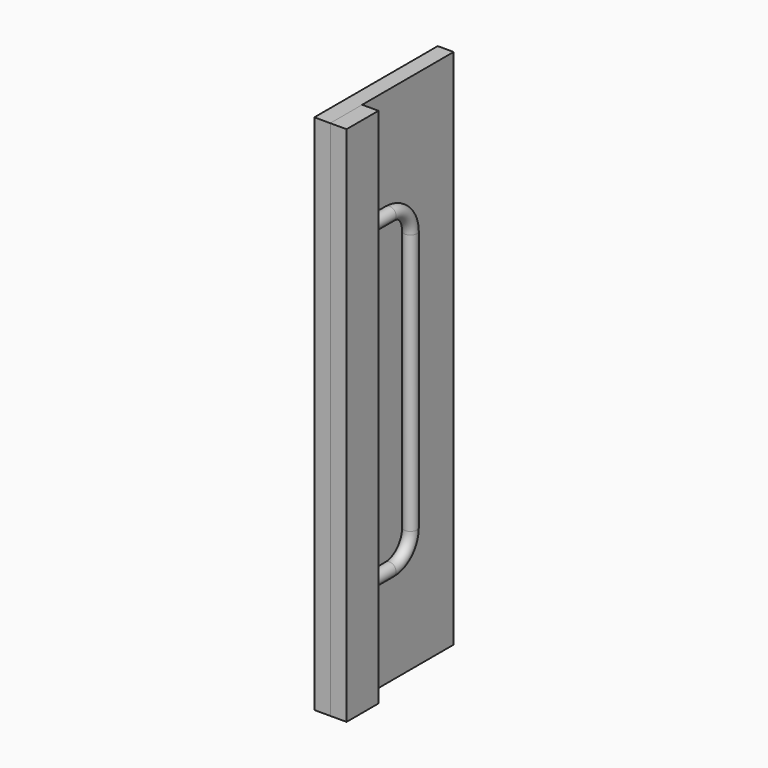
from build123d import *

# Parameters (mm, degrees)
F1_R     = 6.35
F5_DEPTH = 254
F4_W     = 15.4882142484
F4_H     = 150.1632109284
F6_DEPTH = 254


with BuildPart() as f2:
    # F2: sweep along a path in F0
    with BuildLine(Plane.YZ) as f2_path:
        Line((-25.4, 152.4), (0, 152.4))
        ThreePointArc((0, 152.4), (17.9605122421, 144.9605122421), (25.4, 127))
        Line((25.4, 127), (25.4, 0))
        Line((25.4, 0), (25.4, -127))
        ThreePointArc((25.4, -127), (17.9605122421, -144.9605122421), (0, -152.4))
        Line((0, -152.4), (-25.4, -152.4))
    # F1 (on Top) → F2 (sweep)
    with BuildSketch(Plane.XY):
        with Locations((0, 25.4)):
            Circle(F1_R)
    sweep(path=f2_path.line)


with BuildPart() as f5:
    # F3 (on Top) → F5 (new body, symmetric)
    with BuildSketch(Plane.XY):
        Polygon((9.525, -25.4), (6.35, -25.4), (-6.35, -25.4), (-6.35, -64.2415359616), (9.525, -64.2415359616), align=None)
    extrude(amount=F5_DEPTH, both=True)


with BuildPart() as f6:
    # F4 (on Top) → F6 (new body, symmetric)
    with BuildSketch(Plane.XY):
        with Locations((-14.0941071242, 10.8400695026)):
            Rectangle(F4_W, F4_H)
    extrude(amount=F6_DEPTH, both=True)


solid = Compound([f2.part, f5.part, f6.part])
